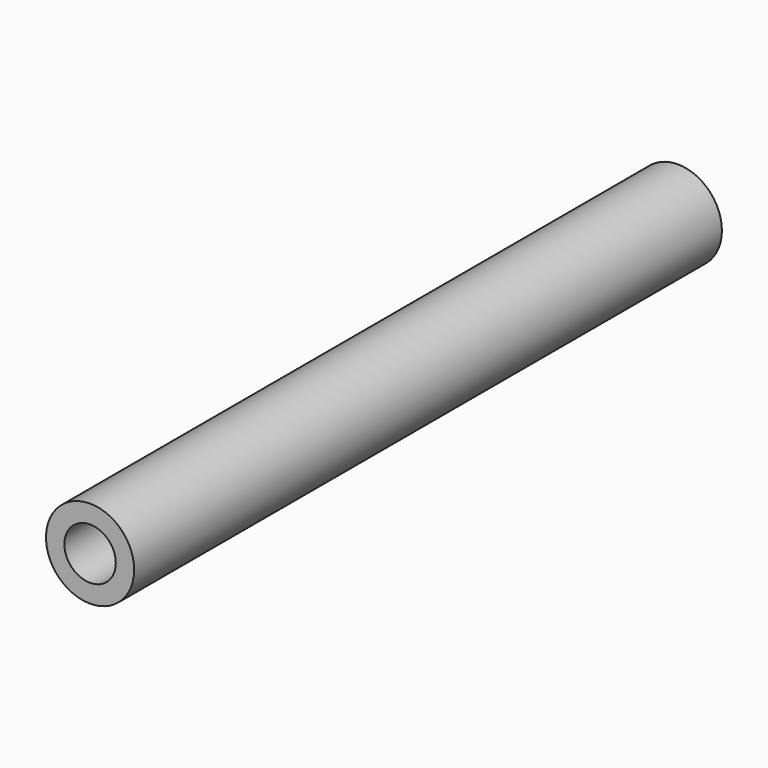
from build123d import *

# Parameters (mm, degrees)
F0_R     = 60
F0_R_2   = 35
F1_DEPTH = 1000


# Not quite as in the source:
# - a feature of the source that left no trace in its solid (it failed there, or was rolled back) is left out
# - the program builds the solid bodies; features that only make, move or delete a surface that nothing else refers to are left out


with BuildPart() as f1:
    # F0 (on Front) → F1 (new body)
    with BuildSketch(Plane.XZ):
        Circle(F0_R)
        Circle(F0_R_2, mode=Mode.SUBTRACT)
    extrude(amount=F1_DEPTH)


solid = f1.part
